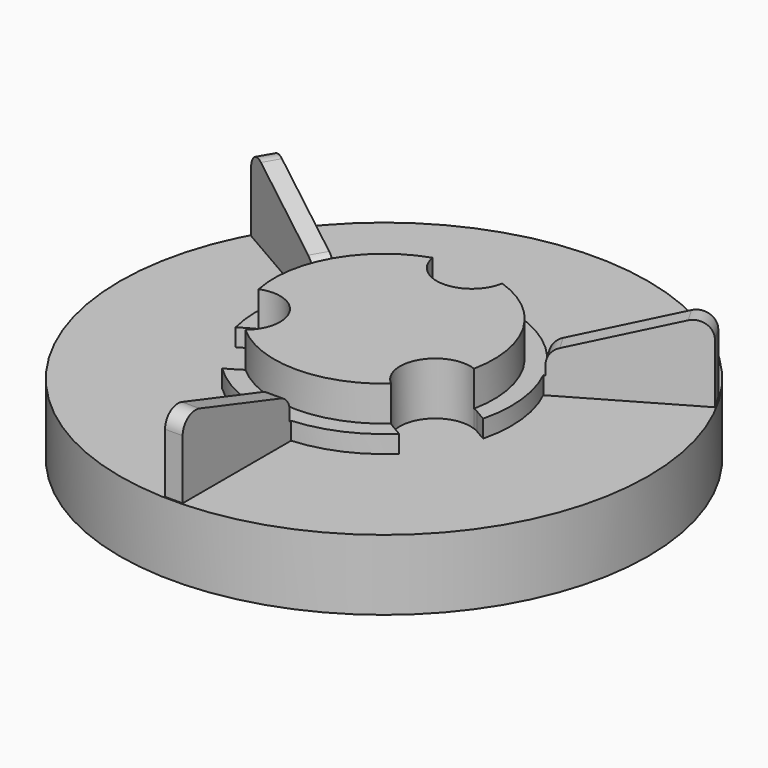
from build123d import *

# Parameters (mm, degrees)
F0_R            = 47.625
F1_DEPTH        = 12.7
F2_R            = 19.812
F3_DEPTH        = 9.525
F4_R            = 22.987
F4_R_2          = 19.812
F5_DEPTH        = 3.175
F7_DEPTH        = 9.525
F9_DEPTH        = 1.5875
F9_COPIES_COUNT = 3


# Not quite as in the source:
# - a pattern or mirror of a feature is missing from the dataset's text; its kind, count and spacing are read off the source's solid


with BuildPart() as f1:
    # F0 (on Top) → F1 (new body)
    with BuildSketch(Plane.XY):
        Circle(F0_R)
    extrude(amount=F1_DEPTH)

    # F2 (on face) → F3 (join)
    with BuildSketch(Plane.XY.offset(12.7)):
        Circle(F2_R)
    extrude(amount=F3_DEPTH)

    # F4 (on face) → F5 (join)
    with BuildSketch(Plane.XY.offset(12.7)):
        Circle(F4_R)
        Circle(F4_R_2, mode=Mode.SUBTRACT)
    extrude(amount=F5_DEPTH)

    # F6 (on face) → F7 (cut, through all)
    with BuildSketch(Plane.XY.offset(22.225)):
        with BuildLine():
            Line((22.307688043, -5.5470012779), (20.3326952998, -4.406738686))
            ThreePointArc((20.3326952998, -4.406738686), (19.8803431182, -4.1693033149), (19.4103678781, -3.9690002312))
            ThreePointArc((19.4103678781, -3.9690002312), (17.1576952998, -9.906), (13.1424389669, -14.8253715637))
            ThreePointArc((13.1424389669, -14.8253715637), (13.5508941459, -15.1322305189), (13.9826952998, -15.405261314))
            Line((13.9826952998, -15.405261314), (15.957688043, -16.545523906))
            ThreePointArc((15.957688043, -16.545523906), (19.9073259568, -11.4935), (22.307688043, -5.5470012779))
        make_face()
        with BuildLine():
            ThreePointArc((13.1424389669, -14.8253715637), (17.1576952998, -9.906), (19.4103678781, -3.9690002312))
            ThreePointArc((19.4103678781, -3.9690002312), (11.6584339857, -6.731), (13.1424389669, -14.8253715637))
        make_face()
        with BuildLine():
            ThreePointArc((-13.9826952998, -15.405261314), (-13.5508941459, -15.1322305189), (-13.1424389669, -14.8253715637))
            ThreePointArc((-13.1424389669, -14.8253715637), (-17.1576952998, -9.906), (-19.4103678781, -3.9690002312))
            ThreePointArc((-19.4103678781, -3.9690002312), (-19.8803431182, -4.1693033149), (-20.3326952998, -4.406738686))
            Line((-20.3326952998, -4.406738686), (-22.307688043, -5.5470012779))
            ThreePointArc((-22.307688043, -5.5470012779), (-19.9073259568, -11.4935), (-15.957688043, -16.545523906))
            Line((-15.957688043, -16.545523906), (-13.9826952998, -15.405261314))
        make_face()
        with BuildLine():
            ThreePointArc((-19.4103678781, -3.9690002312), (-17.1576952998, -9.906), (-13.1424389669, -14.8253715637))
            ThreePointArc((-13.1424389669, -14.8253715637), (-11.6584339857, -6.731), (-19.4103678781, -3.9690002312))
        make_face()
        with BuildLine():
            ThreePointArc((-6.2679289112, 18.7943717949), (0, 13.462), (6.2679289112, 18.7943717949))
            ThreePointArc((6.2679289112, 18.7943717949), (0, 19.812), (-6.2679289112, 18.7943717949))
        make_face()
        with BuildLine():
            ThreePointArc((-6.2679289112, 18.7943717949), (0, 19.812), (6.2679289112, 18.7943717949))
            ThreePointArc((6.2679289112, 18.7943717949), (6.3294489723, 19.3015338338), (6.35, 19.812))
            Line((6.35, 19.812), (6.35, 22.0925251839))
            ThreePointArc((6.35, 22.0925251839), (0, 22.987), (-6.35, 22.0925251839))
            Line((-6.35, 22.0925251839), (-6.35, 19.812))
            ThreePointArc((-6.35, 19.812), (-6.3294489723, 19.3015338338), (-6.2679289112, 18.7943717949))
        make_face()
    extrude(amount=-F7_DEPTH, mode=Mode.SUBTRACT)

    # F8 (on Right) → F9 (join, symmetric)
    with BuildSketch(Plane.YZ):
        with BuildLine():
            Line((-21.5231496841, 11.5825022791), (-21.5231496841, 15.875))
            Line((-21.5231496841, 15.875), (-23.241, 15.875))
            Line((-23.241, 15.875), (-23.241, 17.5747702103))
            ThreePointArc((-23.241, 17.5747702103), (-23.8028498992, 19.2971673195), (-25.2722576527, 20.3569635098))
            Line((-25.2722576527, 20.3569635098), (-43.5602576527, 26.2054457308))
            ThreePointArc((-43.5602576527, 26.2054457308), (-46.1723971092, 25.7824025322), (-47.371, 23.4232524314))
            Line((-47.371, 23.4232524314), (-47.371, 11.5825022791))
            Line((-47.371, 11.5825022791), (-21.5231496841, 11.5825022791))
        make_face()
    f9 = extrude(amount=F9_DEPTH, both=True)

    # F9_copies: F9 ×3 about axis
    f9_copies_axis = Axis((0, 0, 0), (0, 0, 1))
    for i in range(1, F9_COPIES_COUNT):
        add(f9.rotate(f9_copies_axis, i * 360 / F9_COPIES_COUNT))


solid = f1.part
